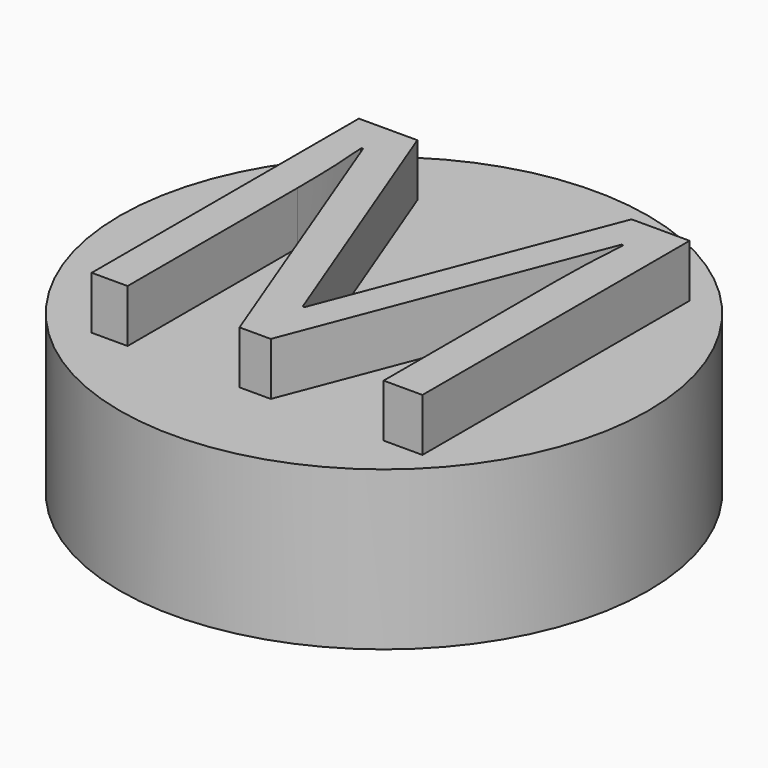
from build123d import *

# Parameters (mm, degrees)
F0_R         = 5
F1_DEPTH     = 3
F2_TEXT_SIZE = 8.8551071394
F3_DEPTH     = 1


# Not quite as in the source:
# - Text() gives the source's letters only with a copy of the font that has no kerning and outlines rounded to 1/6400 em; it was checked with that copy


with BuildPart() as f1:
    # F0 (on Top) → F1 (new body)
    with BuildSketch(Plane.XY):
        Circle(F0_R)
    extrude(amount=F1_DEPTH)

    # F2 (on face) → F3 (join)
    with BuildSketch(Plane.XY.offset(3)):
        with Locations((-3.8519716056, -3.1878385702)):
            Text('M', F2_TEXT_SIZE, font='Open Sans', text_align=(TextAlign.LEFT, TextAlign.BOTTOM))
    extrude(amount=F3_DEPTH)


solid = f1.part
